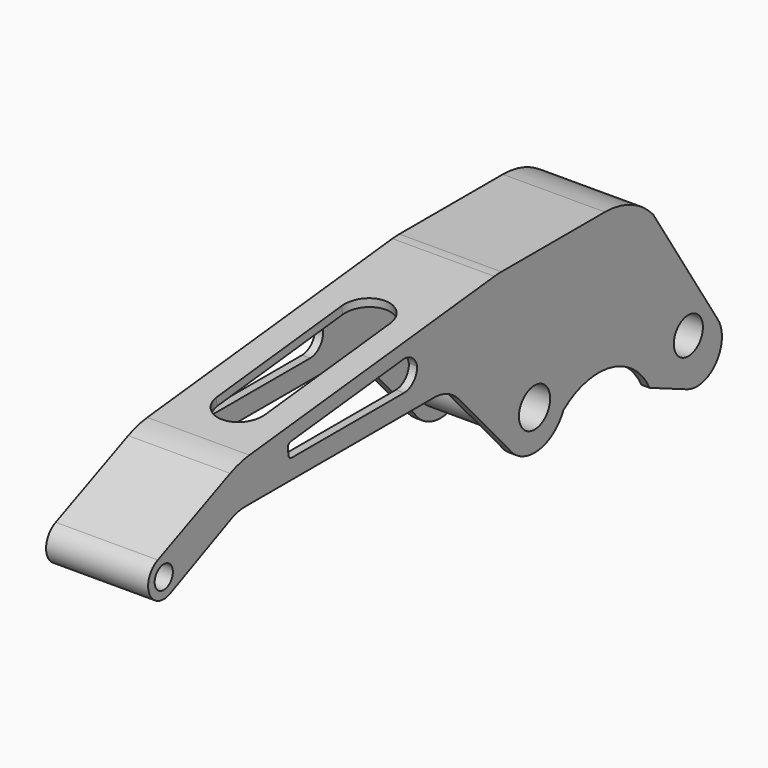
from build123d import *

# Parameters (mm, degrees)
F0_R        = 5.6533409101
F0_R_2      = 6.0582147302
F0_R_3      = 3.5468264326
F1_DEPTH    = 31.75
F2_T        = 2.54
F2_T3_DEPTH = 36.83
F4_DEPTH    = 25.4
F6_DEPTH    = 31.751
F7_T1_DEPTH = 2.54
F7_T3_DEPTH = 2.54
F8_R        = 1.27


# Not quite as in the source:
# - a fillet or chamfer that OpenCascade refuses, or shapes differently, is made with other operations: its cross-section is extruded or revolved along the edge and cut away or added
# - a shell that OpenCascade refuses in one call is made with other operations: the cavity is built on its own and cut out


with BuildPart() as f1:
    # F0 (on Right) → F1 (new body)
    with BuildSketch(Plane.YZ):
        with BuildLine():
            Line((-118.2969192854, 30.0553025028), (-146.4621126652, 17.7829619497))
            ThreePointArc((-146.4621126652, 17.7829619497), (-149.6721200055, 9.657338463), (-141.4359788777, 6.7425685756))
            Line((-141.4359788777, 6.7425685756), (-117.9046317908, 17.455203049))
            ThreePointArc((-117.9046317908, 17.455203049), (-115.3347971308, 18.3079832041), (-112.6425907814, 18.5966164392))
            Line((-112.6425907814, 18.5966164392), (-39.032237408, 18.5966164392))
            ThreePointArc((-39.032237408, 18.5966164392), (-33.875711062, 17.5026595222), (-29.6075339545, 14.4092520366))
            Line((-29.6075339545, 14.4092520366), (-10.1635284412, -7.1180392256))
            ThreePointArc((-10.1635284412, -7.1180392256), (1.0358015594, -12.3649063046), (11.2061193672, -5.3279153072))
            ThreePointArc((11.2061193672, -5.3279153072), (29.7519512617, -1.1293262164), (44.7507215315, -12.8174792531))
            Line((44.7507215315, -12.8174792531), (59.2673632914, -19.1176440206))
            ThreePointArc((59.2673632914, -19.1176440206), (70.5449926496, -16.490786447), (71.3009120761, -4.9359653548))
            Line((71.3009120761, -4.9359653548), (46.0699528524, 34.1704526075))
            ThreePointArc((46.0699528524, 34.1704526075), (37.5779975797, 40.2467968073), (27.3589767296, 42.3931602559))
            Line((27.3589767296, 42.3931602559), (-12.8688071267, 42.3931602559))
            ThreePointArc((-12.8688071267, 42.3931602559), (-14.2256285087, 42.3568949126), (-15.5785754345, 42.2482024399))
            Line((-15.5785754345, 42.2482024399), (-110.8605493232, 32.0248153133))
            ThreePointArc((-110.8605493232, 32.0248153133), (-114.6537287056, 31.3232183323), (-118.2969192854, 30.0553025028))
        make_face()
        with Locations((59.7972124815, -4.6163224615)):
            Circle(F0_R, mode=Mode.SUBTRACT)
        Circle(F0_R_2, mode=Mode.SUBTRACT)
        with Locations((-144.1483274102, 12.1720423922)):
            Circle(F0_R_3, mode=Mode.SUBTRACT)
    extrude(amount=F1_DEPTH)

    # F2: shell of thickness 2.54, made by hand


with BuildPart() as f2_core1:
    # F2_t2: copy of F1
    add(f1.part)

    # the walls: a layer under each face that stays
    f2_faces = [f2_core1.faces().sort_by_distance(p)[0] for p in [
        (15.875, -63.2195623789, 37.1365088766),
        (15.875, -114.6537287056, 31.3232183323),
        (15.875, -132.3795159753, 23.9191322262),
        (15.875, -149.6721200055, 9.657338463),
        (15.875, 58.6854324642, 14.6172436263),
        (15.875, 37.5779975797, 40.2467968073),
        (15.875, 7.2450848014, 42.3931602559),
        (15.875, -14.2256285087, 42.3568949126),
        (15.875, 54.1438715714, -4.6163224615),
        (15.875, -6.0582147302, 0),
        (15.875, -147.6951538428, 12.1720423922),
        (0, -38.6823777389, 32.0074819355),
        (31.75, -38.6823777389, 32.0074819355),
    ]]
    thicken(f2_faces, amount=-F2_T, mode=Mode.SUBTRACT)

    # F2_s4 → F2_t3 (cut)
    with BuildSketch(Plane.YZ.offset(-2.54)):
        Polygon((-146.4819420371, 17.8297292802), (-145.4474988382, 15.4544090123), (-145.4705469322, 15.4443663311), (-145.4937892966, 15.4347818344), align=None)
    extrude(amount=F2_T3_DEPTH, mode=Mode.SUBTRACT)


with BuildPart() as f1_1:
    add(f1.part)

    # what is left inside the walls is the cavity
    f2_cavity = [f2_core1.part.solids().sort_by_distance(p)[0] for p in [
        (29.1846, -87.664257, 19.92847),
    ]]
    add(f2_cavity, mode=Mode.SUBTRACT)

    # F3 (on face) → F4 (cut)
    with BuildSketch(Plane(origin=(0, -4.6587823298, 43.4198539884), x_dir=(1, 0, 0), z_dir=(0, -0.1066837916, 0.9942929994))):
        with BuildLine():
            Line((8.5797651154, -41.550964987), (8.5891456531, -90.6220046018))
            ThreePointArc((8.5891456531, -90.6220046018), (15.9863896259, -97.7322088228), (23.5313536211, -90.7789548531))
            Line((23.5313536211, -90.7789548531), (23.5313536211, -42.0811111897))
            ThreePointArc((23.5313536211, -42.0811111897), (16.3302504196, -34.0689910553), (8.5797651154, -41.550964987))
        make_face()
    extrude(amount=-F4_DEPTH, mode=Mode.SUBTRACT)

    # F5 (on face) → F6 (cut, through all)
    with BuildSketch(Plane.YZ.offset(31.75)):
        Polygon((-46.1267865209, 34.4621779106), (-96.0500612855, 29.1056036949), (-95.512650907, 24.6252825343), (-45.0713257087, 24.6252825343), align=None)
    extrude(amount=-F6_DEPTH, mode=Mode.SUBTRACT)

    # F7: fillet of radius 5.08 on 4 edges, made by hand

    # F7_s2 → F7_t1 (join)
    with BuildSketch(Plane.YZ.offset(29.21)):
        with BuildLine():
            ThreePointArc((-50.7255480205, 24.6252825343), (-46.9466907461, 26.3101922999), (-45.6745395837, 30.2472361958))
            Line((-45.6745395837, 30.2472361958), (-45.0713257087, 24.6252825343))
            Line((-45.0713257087, 24.6252825343), (-50.7255480205, 24.6252825343))
        make_face()
        with BuildLine():
            ThreePointArc((-51.1777949577, 33.920224249), (-47.4474580879, 32.8240372389), (-45.5848328594, 29.4111694737))
            Line((-45.5848328594, 29.4111694737), (-46.1267865209, 34.4621779106))
            Line((-46.1267865209, 34.4621779106), (-51.1777949577, 33.920224249))
        make_face()
    extrude(amount=F7_T1_DEPTH)

    # F7_s4 → F7_t3 (join)
    with BuildSketch(Plane.YZ):
        with BuildLine():
            ThreePointArc((-51.1777949577, 33.920224249), (-47.4474580879, 32.8240372389), (-45.5848328594, 29.4111694737))
            Line((-45.5848328594, 29.4111694737), (-46.1267865209, 34.4621779106))
            Line((-46.1267865209, 34.4621779106), (-51.1777949577, 33.920224249))
        make_face()
        with BuildLine():
            ThreePointArc((-50.7255480205, 24.6252825343), (-46.9466907461, 26.3101922999), (-45.6745395837, 30.2472361958))
            Line((-45.6745395837, 30.2472361958), (-45.0713257087, 24.6252825343))
            Line((-45.0713257087, 24.6252825343), (-50.7255480205, 24.6252825343))
        make_face()
    extrude(amount=F7_T3_DEPTH)

    # F8
    f8_edges = [f1_1.edges().sort_by_distance(p)[0] for p in [
        (30.48, -96.050061, 29.105604),
        (30.48, -95.512651, 24.625283),
        (1.27, -96.050061, 29.105604),
        (1.27, -95.512651, 24.625283),
    ]]
    fillet(f8_edges, radius=F8_R)


solid = f1_1.part
